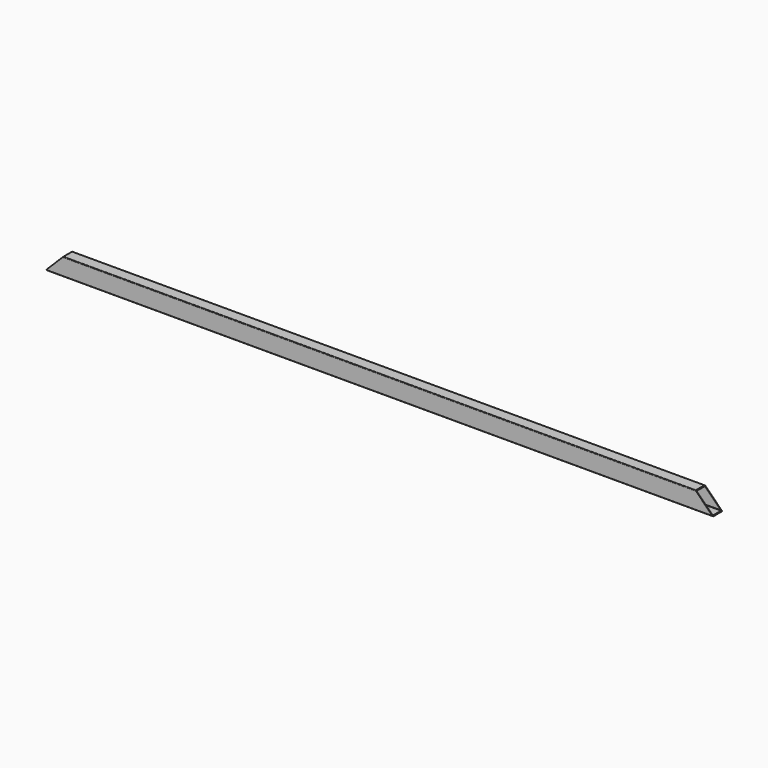
from build123d import *

# Parameters (mm, degrees)
F1_DEPTH      = 1150
F1_DEPTH_BACK = 1150
F3_DEPTH      = 25
F3_DEPTH_BACK = 25


with BuildPart() as f1:
    # F0 (on Right) → F1 (new body, two sides)
    with BuildSketch(Plane.YZ) as f1_sk:
        with BuildLine():
            ThreePointArc((-20, -28), (-19.4142135624, -29.4142135624), (-18, -30))
            Line((-18, -30), (18, -30))
            ThreePointArc((18, -30), (19.4142135624, -29.4142135624), (20, -28))
            Line((20, -28), (20, 28))
            ThreePointArc((20, 28), (19.4142135624, 29.4142135624), (18, 30))
            Line((18, 30), (-18, 30))
            ThreePointArc((-18, 30), (-19.4142135624, 29.4142135624), (-20, 28))
            Line((-20, 28), (-20, -28))
        make_face()
        with BuildLine():
            Line((17, -28), (-17, -28))
            ThreePointArc((-17, -28), (-17.7071067812, -27.7071067812), (-18, -27))
            Line((-18, -27), (-18, 27))
            ThreePointArc((-18, 27), (-17.7071067812, 27.7071067812), (-17, 28))
            Line((-17, 28), (17, 28))
            ThreePointArc((17, 28), (17.7071067812, 27.7071067812), (18, 27))
            Line((18, 27), (18, -27))
            ThreePointArc((18, -27), (17.7071067812, -27.7071067812), (17, -28))
        make_face(mode=Mode.SUBTRACT)
    extrude(amount=F1_DEPTH)
    extrude(f1_sk.sketch, amount=-F1_DEPTH_BACK)

    # F2 (on Front) → F3 (cut, two sides)
    with BuildSketch(Plane.XZ) as f3_sk:
        Polygon((-1150, 30), (-1150, -30), (-1090, 30), align=None)
        Polygon((1090, 30), (1150, -30), (1150, 30), align=None)
    extrude(amount=-F3_DEPTH, mode=Mode.SUBTRACT)
    extrude(f3_sk.sketch, amount=F3_DEPTH_BACK, mode=Mode.SUBTRACT)


solid = f1.part
